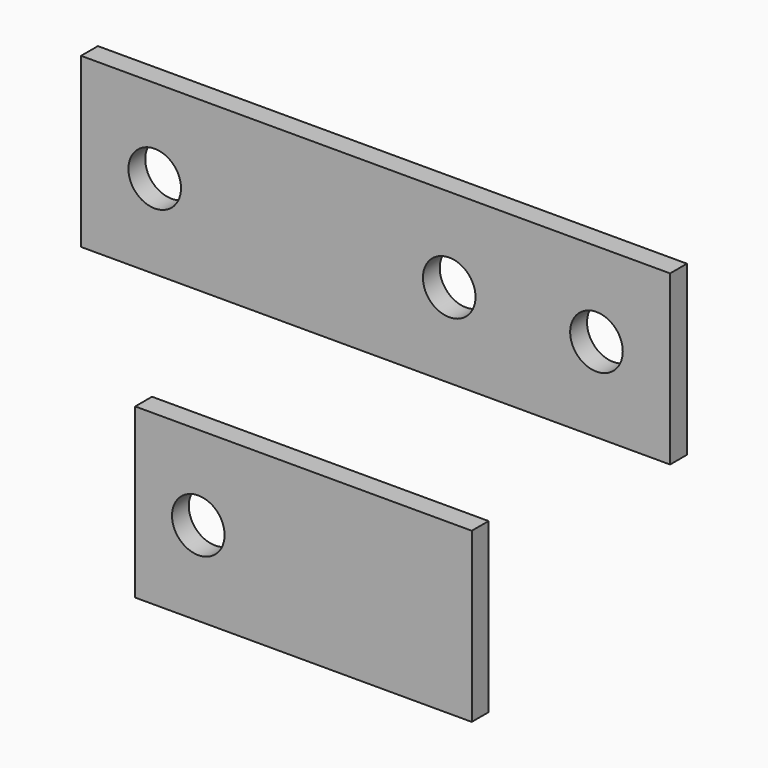
from build123d import *

# Parameters (mm, degrees)
F0_W     = 88.9
F0_H     = 25.4
F1_DEPTH = 3.175
F0_W_2   = 50.8
F2_R     = 3.96875
F3_DEPTH = 3.176


# Not quite as in the source:
# - a feature names something its author has since deleted; it is built from what else it names


with BuildPart() as f1:
    # F0 (on Front) → F1 (new body)
    with BuildSketch(Plane.XZ):
        with Locations((-17.0495061394, 46.5531354078)):
            Rectangle(F0_W, F0_H)
    extrude(amount=F1_DEPTH)


with BuildPart() as f1b:
    # F0 (on Front) → F1, piece 2 (new body)
    with BuildSketch(Plane.XZ):
        with Locations((-27.9352209627, 2.6215043573)):
            Rectangle(F0_W_2, F0_H)
    extrude(amount=F1_DEPTH)


with BuildPart() as f3_tool:
    # F2 (on face) → F3 (new body, through all)
    with BuildSketch(Plane.XZ.offset(3.175)):
        with Locations((-50.3870061394, 46.5531354078)):
            Circle(F2_R)
        with Locations((-43.8102209627, 2.6215043573)):
            Circle(F2_R)
        with Locations((-5.9370061394, 46.5531354078)):
            Circle(F2_R)
        with Locations((16.2879938606, 46.5531354078)):
            Circle(F2_R)
    extrude(amount=-F3_DEPTH)


with BuildPart() as f1_1:
    add(f1.part)

    # F3: cut by f3_tool
    add(f3_tool.part, mode=Mode.SUBTRACT)


with BuildPart() as f1b_1:
    add(f1b.part)

    # F3: cut by f3_tool
    add(f3_tool.part, mode=Mode.SUBTRACT)


solid = Compound([f1_1.part, f1b_1.part])
